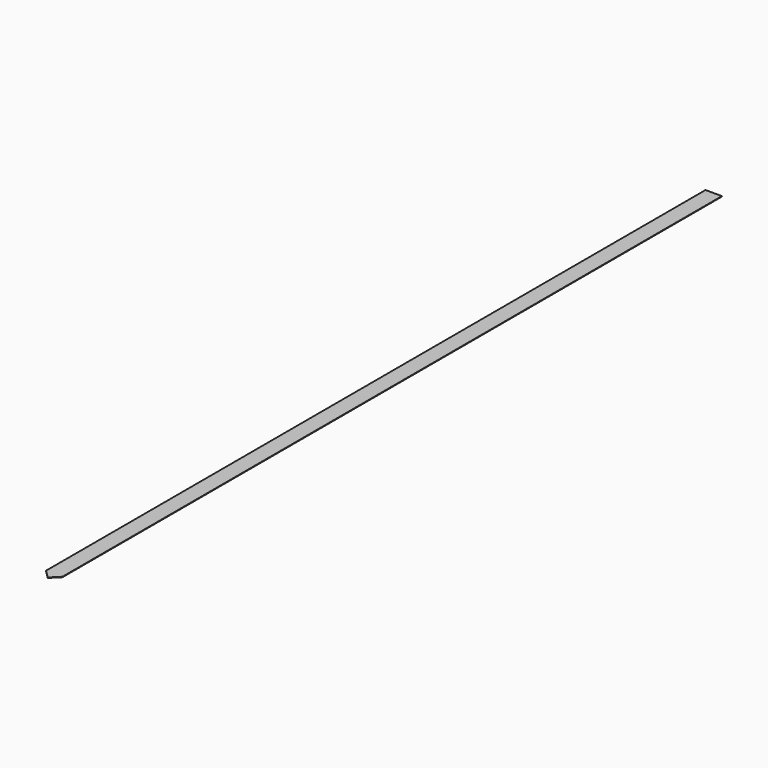
from build123d import *

# Parameters (mm, degrees)
F0_W        = 79.1414380074
F0_H        = 2.1752845496
F1_DEPTH    = 4010
F2_T1_DEPTH = 207.9099235869


# Not quite as in the source:
# - a fillet or chamfer that OpenCascade refuses, or shapes differently, is made with other operations: its cross-section is extruded or revolved along the edge and cut away or added


with BuildPart() as f1:
    # F0 (on Front) → F1 (new body)
    with BuildSketch(Plane.XZ):
        Rectangle(F0_W, F0_H)
    extrude(amount=F1_DEPTH)

    # F2: chamfer of 40 on 2 edges, made by hand

    # F2_s2 → F2_t1 (cut)
    with BuildSketch(Plane.XY.offset(-103.9549617934)):
        Polygon((39.5707190037, -3970), (-0.4292809963, -4010), (39.5707190037, -4010), align=None)
        Polygon((-39.5707190037, -3970), (0.4292809963, -4010), (-39.5707190037, -4010), align=None)
    extrude(amount=F2_T1_DEPTH, mode=Mode.SUBTRACT)


solid = f1.part
